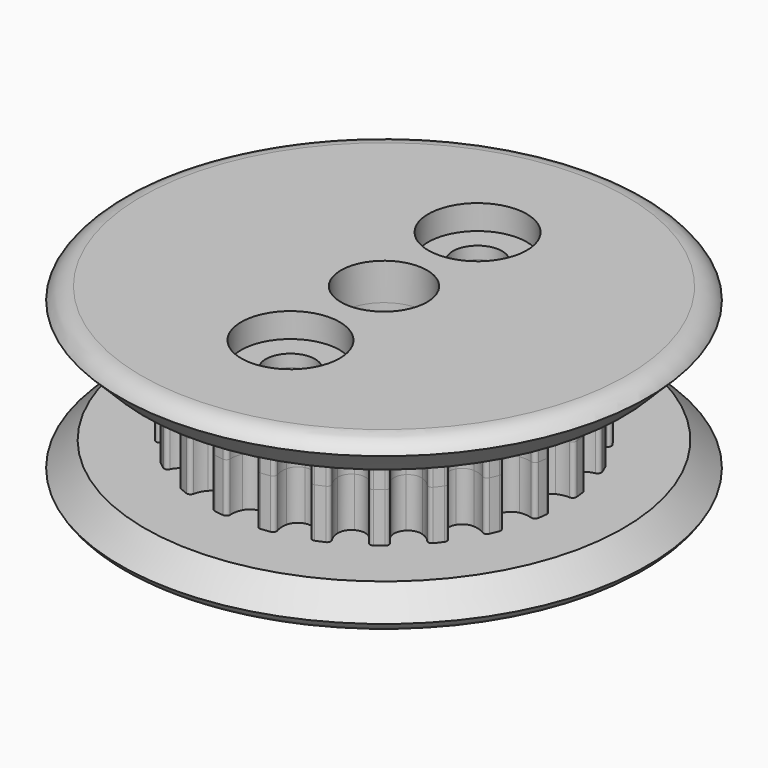
from build123d import *

# Parameters (mm, degrees)
F1_DEPTH      = 2
F1_DEPTH_BACK = 2
F4_SIZE       = 1
F4_2_SIZE     = 1
F6_R          = 1.75
F6_R_2        = 1
F7_DEPTH      = 7.001
F8_R          = 2
F9_DEPTH      = 1


# Not quite as in the source:
# - a fillet or chamfer that OpenCascade refuses, or shapes differently, is made with other operations: its cross-section is extruded or revolved along the edge and cut away or added


with BuildPart() as f1:
    # F0 (on Top) → F1 (new body, two sides)
    with BuildSketch(Plane.XY) as f1_sk:
        with BuildLine():
            ThreePointArc((-0.5986152965, 7.0620442035), (-0.6451801887, 7.1787658618), (-0.7641980304, 7.2191018018))
            ThreePointArc((-0.7641980304, 7.2191018018), (-0.9475467043, 7.1973317762), (-1.1302824209, 7.1709058774))
            ThreePointArc((-1.1302824209, 7.1709058774), (-1.2348051185, 7.1011402672), (-1.2495735623, 6.976343922))
            ThreePointArc((-1.2495735623, 6.976343922), (-1.2024254376, 6.7283466079), (-1.2188831701, 6.4764443322))
            ThreePointArc((-1.2188831701, 6.4764443322), (-1.3577692814, 6.2037699974), (-1.6200615767, 6.0461521156))
            ThreePointArc((-1.6200615767, 6.0461521156), (-1.9260223085, 6.0515070577), (-2.1826383766, 6.218206903))
            ThreePointArc((-2.1826383766, 6.218206903), (-2.3228423289, 6.4281318067), (-2.4060095121, 6.6664778432))
            ThreePointArc((-2.4060095121, 6.6664778432), (-2.4811975322, 6.7671704264), (-2.6065996488, 6.7753278684))
            ThreePointArc((-2.6065996488, 6.7753278684), (-2.7780663709, 6.7068455098), (-2.947735993, 6.634024568))
            ThreePointArc((-2.947735993, 6.634024568), (-3.0306404975, 6.5395836985), (-3.0126060479, 6.4152173311))
            ThreePointArc((-3.0126060479, 6.4152173311), (-2.9028780285, 6.1878731533), (-2.853577871, 5.9402946649))
            ThreePointArc((-2.853577871, 5.9402946649), (-2.9171582418, 5.6409651119), (-3.1297186342, 5.4208316878))
            ThreePointArc((-3.1297186342, 5.4208316878), (-3.4266399679, 5.3468157002), (-3.7176571503, 5.4414182604))
            ThreePointArc((-3.7176571503, 5.4414182604), (-3.9074163319, 5.6079026934), (-4.0494381556, 5.8166020346))
            ThreePointArc((-4.0494381556, 5.8166020346), (-4.1481253643, 5.8944035098), (-4.2713658087, 5.8698265376))
            ThreePointArc((-4.2713658087, 5.8698265376), (-4.4192654053, 5.7592988055), (-4.5643062286, 5.6450454476))
            ThreePointArc((-4.5643062286, 5.6450454476), (-4.6199427349, 5.5323653079), (-4.5703344099, 5.4169042808))
            ThreePointArc((-4.5703344099, 5.4169042808), (-4.4055042791, 5.2257063691), (-4.2938059557, 4.9993237329))
            ThreePointArc((-4.2938059557, 4.9993237329), (-4.2777476889, 4.6937377762), (-4.4260905389, 4.4260905389))
            ThreePointArc((-4.4260905389, 4.4260905389), (-4.6937377762, 4.2777476889), (-4.9993237329, 4.2938059557))
            ThreePointArc((-4.9993237329, 4.2938059557), (-5.2257063691, 4.4055042791), (-5.4169042808, 4.5703344099))
            ThreePointArc((-5.4169042808, 4.5703344099), (-5.5323653079, 4.6199427349), (-5.6450454476, 4.5643062286))
            ThreePointArc((-5.6450454476, 4.5643062286), (-5.7592988055, 4.4192654053), (-5.8698265376, 4.2713658087))
            ThreePointArc((-5.8698265376, 4.2713658087), (-5.8944035098, 4.1481253643), (-5.8166020346, 4.0494381556))
            ThreePointArc((-5.8166020346, 4.0494381556), (-5.6079026934, 3.9074163319), (-5.4414182604, 3.7176571503))
            ThreePointArc((-5.4414182604, 3.7176571503), (-5.3468157002, 3.4266399679), (-5.4208316878, 3.1297186342))
            ThreePointArc((-5.4208316878, 3.1297186342), (-5.6409651119, 2.9171582418), (-5.9402946649, 2.853577871))
            ThreePointArc((-5.9402946649, 2.853577871), (-6.1878731533, 2.9028780285), (-6.4152173311, 3.0126060479))
            ThreePointArc((-6.4152173311, 3.0126060479), (-6.5395836985, 3.0306404975), (-6.634024568, 2.947735993))
            ThreePointArc((-6.634024568, 2.947735993), (-6.7068455098, 2.7780663709), (-6.7753278684, 2.6065996488))
            ThreePointArc((-6.7753278684, 2.6065996488), (-6.7671704264, 2.4811975322), (-6.6664778432, 2.4060095121))
            ThreePointArc((-6.6664778432, 2.4060095121), (-6.4281318067, 2.3228423289), (-6.218206903, 2.1826383766))
            ThreePointArc((-6.218206903, 2.1826383766), (-6.0515070577, 1.9260223085), (-6.0461521156, 1.6200615767))
            ThreePointArc((-6.0461521156, 1.6200615767), (-6.2037699974, 1.3577692814), (-6.4764443322, 1.2188831701))
            ThreePointArc((-6.4764443322, 1.2188831701), (-6.7283466079, 1.2024254376), (-6.976343922, 1.2495735623))
            ThreePointArc((-6.976343922, 1.2495735623), (-7.1011402672, 1.2348051185), (-7.1709058774, 1.1302824209))
            ThreePointArc((-7.1709058774, 1.1302824209), (-7.1973317762, 0.9475467043), (-7.2191018018, 0.7641980304))
            ThreePointArc((-7.2191018018, 0.7641980304), (-7.1787658618, 0.6451801887), (-7.0620442035, 0.5986152965))
            ThreePointArc((-7.0620442035, 0.5986152965), (-6.8102943604, 0.5799704599), (-6.5712350212, 0.4988764045))
            ThreePointArc((-6.5712350212, 0.4988764045), (-6.3437982097, 0.2941494117), (-6.2594372684, 0))
            ThreePointArc((-6.2594372684, 0), (-6.3437982097, -0.2941494117), (-6.5712350212, -0.4988764045))
            ThreePointArc((-6.5712350212, -0.4988764045), (-6.8102943604, -0.5799704599), (-7.0620442035, -0.5986152965))
            ThreePointArc((-7.0620442035, -0.5986152965), (-7.1787658618, -0.6451801887), (-7.2191018018, -0.7641980304))
            ThreePointArc((-7.2191018018, -0.7641980304), (-7.1973317762, -0.9475467043), (-7.1709058774, -1.1302824209))
            ThreePointArc((-7.1709058774, -1.1302824209), (-7.1011402672, -1.2348051185), (-6.976343922, -1.2495735623))
            ThreePointArc((-6.976343922, -1.2495735623), (-6.7283466079, -1.2024254376), (-6.4764443322, -1.2188831701))
            ThreePointArc((-6.4764443322, -1.2188831701), (-6.2037699974, -1.3577692814), (-6.0461521156, -1.6200615767))
            ThreePointArc((-6.0461521156, -1.6200615767), (-6.0515070577, -1.9260223085), (-6.218206903, -2.1826383766))
            ThreePointArc((-6.218206903, -2.1826383766), (-6.4281318067, -2.3228423289), (-6.6664778432, -2.4060095121))
            ThreePointArc((-6.6664778432, -2.4060095121), (-6.7671704264, -2.4811975322), (-6.7753278684, -2.6065996488))
            ThreePointArc((-6.7753278684, -2.6065996488), (-6.7068455098, -2.7780663709), (-6.634024568, -2.947735993))
            ThreePointArc((-6.634024568, -2.947735993), (-6.5395836985, -3.0306404975), (-6.4152173311, -3.0126060479))
            ThreePointArc((-6.4152173311, -3.0126060479), (-6.1878731533, -2.9028780285), (-5.9402946649, -2.853577871))
            ThreePointArc((-5.9402946649, -2.853577871), (-5.6409651119, -2.9171582418), (-5.4208316878, -3.1297186342))
            ThreePointArc((-5.4208316878, -3.1297186342), (-5.3468157002, -3.4266399679), (-5.4414182604, -3.7176571503))
            ThreePointArc((-5.4414182604, -3.7176571503), (-5.6079026934, -3.9074163319), (-5.8166020346, -4.0494381556))
            ThreePointArc((-5.8166020346, -4.0494381556), (-5.8944035098, -4.1481253643), (-5.8698265376, -4.2713658087))
            ThreePointArc((-5.8698265376, -4.2713658087), (-5.7592988055, -4.4192654053), (-5.6450454476, -4.5643062286))
            ThreePointArc((-5.6450454476, -4.5643062286), (-5.5323653079, -4.6199427349), (-5.4169042808, -4.5703344099))
            ThreePointArc((-5.4169042808, -4.5703344099), (-5.2257063691, -4.4055042791), (-4.9993237329, -4.2938059557))
            ThreePointArc((-4.9993237329, -4.2938059557), (-4.6937377762, -4.2777476889), (-4.4260905389, -4.4260905389))
            ThreePointArc((-4.4260905389, -4.4260905389), (-4.2777476889, -4.6937377762), (-4.2938059557, -4.9993237329))
            ThreePointArc((-4.2938059557, -4.9993237329), (-4.4055042791, -5.2257063691), (-4.5703344099, -5.4169042808))
            ThreePointArc((-4.5703344099, -5.4169042808), (-4.6199427349, -5.5323653079), (-4.5643062286, -5.6450454476))
            ThreePointArc((-4.5643062286, -5.6450454476), (-4.4192654053, -5.7592988055), (-4.2713658087, -5.8698265376))
            ThreePointArc((-4.2713658087, -5.8698265376), (-4.1481253643, -5.8944035098), (-4.0494381556, -5.8166020346))
            ThreePointArc((-4.0494381556, -5.8166020346), (-3.9074163319, -5.6079026934), (-3.7176571503, -5.4414182604))
            ThreePointArc((-3.7176571503, -5.4414182604), (-3.4266399679, -5.3468157002), (-3.1297186342, -5.4208316878))
            ThreePointArc((-3.1297186342, -5.4208316878), (-2.9171582418, -5.6409651119), (-2.853577871, -5.9402946649))
            ThreePointArc((-2.853577871, -5.9402946649), (-2.9028780285, -6.1878731533), (-3.0126060479, -6.4152173311))
            ThreePointArc((-3.0126060479, -6.4152173311), (-3.0306404975, -6.5395836985), (-2.947735993, -6.634024568))
            ThreePointArc((-2.947735993, -6.634024568), (-2.7780663709, -6.7068455098), (-2.6065996488, -6.7753278684))
            ThreePointArc((-2.6065996488, -6.7753278684), (-2.4811975322, -6.7671704264), (-2.4060095121, -6.6664778432))
            ThreePointArc((-2.4060095121, -6.6664778432), (-2.3228423289, -6.4281318067), (-2.1826383766, -6.218206903))
            ThreePointArc((-2.1826383766, -6.218206903), (-1.9260223085, -6.0515070577), (-1.6200615767, -6.0461521156))
            ThreePointArc((-1.6200615767, -6.0461521156), (-1.3577692814, -6.2037699974), (-1.2188831701, -6.4764443322))
            ThreePointArc((-1.2188831701, -6.4764443322), (-1.2024254376, -6.7283466079), (-1.2495735623, -6.976343922))
            ThreePointArc((-1.2495735623, -6.976343922), (-1.2348051185, -7.1011402672), (-1.1302824209, -7.1709058774))
            ThreePointArc((-1.1302824209, -7.1709058774), (-0.9475467043, -7.1973317762), (-0.7641980304, -7.2191018018))
            ThreePointArc((-0.7641980304, -7.2191018018), (-0.6451801887, -7.1787658618), (-0.5986152965, -7.0620442035))
            ThreePointArc((-0.5986152965, -7.0620442035), (-0.5799704599, -6.8102943604), (-0.4988764045, -6.5712350212))
            ThreePointArc((-0.4988764045, -6.5712350212), (-0.2941494117, -6.3437982097), (0, -6.2594372684))
            ThreePointArc((0, -6.2594372684), (0.2941494117, -6.3437982097), (0.4988764045, -6.5712350212))
            ThreePointArc((0.4988764045, -6.5712350212), (0.5799704599, -6.8102943604), (0.5986152965, -7.0620442035))
            ThreePointArc((0.5986152965, -7.0620442035), (0.6451801887, -7.1787658618), (0.7641980304, -7.2191018018))
            ThreePointArc((0.7641980304, -7.2191018018), (0.9475467043, -7.1973317762), (1.1302824209, -7.1709058774))
            ThreePointArc((1.1302824209, -7.1709058774), (1.2348051185, -7.1011402672), (1.2495735623, -6.976343922))
            ThreePointArc((1.2495735623, -6.976343922), (1.2024254376, -6.7283466079), (1.2188831701, -6.4764443322))
            ThreePointArc((1.2188831701, -6.4764443322), (1.3577692814, -6.2037699974), (1.6200615767, -6.0461521156))
            ThreePointArc((1.6200615767, -6.0461521156), (1.9260223085, -6.0515070577), (2.1826383766, -6.218206903))
            ThreePointArc((2.1826383766, -6.218206903), (2.3228423289, -6.4281318067), (2.4060095121, -6.6664778432))
            ThreePointArc((2.4060095121, -6.6664778432), (2.4811975322, -6.7671704264), (2.6065996488, -6.7753278684))
            ThreePointArc((2.6065996488, -6.7753278684), (2.7780663709, -6.7068455098), (2.947735993, -6.634024568))
            ThreePointArc((2.947735993, -6.634024568), (3.0306404975, -6.5395836985), (3.0126060479, -6.4152173311))
            ThreePointArc((3.0126060479, -6.4152173311), (2.9028780285, -6.1878731533), (2.853577871, -5.9402946649))
            ThreePointArc((2.853577871, -5.9402946649), (2.9171582418, -5.6409651119), (3.1297186342, -5.4208316878))
            ThreePointArc((3.1297186342, -5.4208316878), (3.4266399679, -5.3468157002), (3.7176571503, -5.4414182604))
            ThreePointArc((3.7176571503, -5.4414182604), (3.9074163319, -5.6079026934), (4.0494381556, -5.8166020346))
            ThreePointArc((4.0494381556, -5.8166020346), (4.1481253643, -5.8944035098), (4.2713658087, -5.8698265376))
            ThreePointArc((4.2713658087, -5.8698265376), (4.4192654053, -5.7592988055), (4.5643062286, -5.6450454476))
            ThreePointArc((4.5643062286, -5.6450454476), (4.6199427349, -5.5323653079), (4.5703344099, -5.4169042808))
            ThreePointArc((4.5703344099, -5.4169042808), (4.4055042791, -5.2257063691), (4.2938059557, -4.9993237329))
            ThreePointArc((4.2938059557, -4.9993237329), (4.2777476889, -4.6937377762), (4.4260905389, -4.4260905389))
            ThreePointArc((4.4260905389, -4.4260905389), (4.6937377762, -4.2777476889), (4.9993237329, -4.2938059557))
            ThreePointArc((4.9993237329, -4.2938059557), (5.2257063691, -4.4055042791), (5.4169042808, -4.5703344099))
            ThreePointArc((5.4169042808, -4.5703344099), (5.5323653079, -4.6199427349), (5.6450454476, -4.5643062286))
            ThreePointArc((5.6450454476, -4.5643062286), (5.7592988055, -4.4192654053), (5.8698265376, -4.2713658087))
            ThreePointArc((5.8698265376, -4.2713658087), (5.8944035098, -4.1481253643), (5.8166020346, -4.0494381556))
            ThreePointArc((5.8166020346, -4.0494381556), (5.6079026934, -3.9074163319), (5.4414182604, -3.7176571503))
            ThreePointArc((5.4414182604, -3.7176571503), (5.3468157002, -3.4266399679), (5.4208316878, -3.1297186342))
            ThreePointArc((5.4208316878, -3.1297186342), (5.6409651119, -2.9171582418), (5.9402946649, -2.853577871))
            ThreePointArc((5.9402946649, -2.853577871), (6.1878731533, -2.9028780285), (6.4152173311, -3.0126060479))
            ThreePointArc((6.4152173311, -3.0126060479), (6.5395836985, -3.0306404975), (6.634024568, -2.947735993))
            ThreePointArc((6.634024568, -2.947735993), (6.7068455098, -2.7780663709), (6.7753278684, -2.6065996488))
            ThreePointArc((6.7753278684, -2.6065996488), (6.7671704264, -2.4811975322), (6.6664778432, -2.4060095121))
            ThreePointArc((6.6664778432, -2.4060095121), (6.4281318067, -2.3228423289), (6.218206903, -2.1826383766))
            ThreePointArc((6.218206903, -2.1826383766), (6.0515070577, -1.9260223085), (6.0461521156, -1.6200615767))
            ThreePointArc((6.0461521156, -1.6200615767), (6.2037699974, -1.3577692814), (6.4764443322, -1.2188831701))
            ThreePointArc((6.4764443322, -1.2188831701), (6.7283466079, -1.2024254376), (6.976343922, -1.2495735623))
            ThreePointArc((6.976343922, -1.2495735623), (7.1011402672, -1.2348051185), (7.1709058774, -1.1302824209))
            ThreePointArc((7.1709058774, -1.1302824209), (7.1973317762, -0.9475467043), (7.2191018018, -0.7641980304))
            ThreePointArc((7.2191018018, -0.7641980304), (7.1787658618, -0.6451801887), (7.0620442035, -0.5986152965))
            ThreePointArc((7.0620442035, -0.5986152965), (6.8102943604, -0.5799704599), (6.5712350212, -0.4988764045))
            ThreePointArc((6.5712350212, -0.4988764045), (6.3437982097, -0.2941494117), (6.2594372684, 0))
            ThreePointArc((6.2594372684, 0), (6.3437982097, 0.2941494117), (6.5712350212, 0.4988764045))
            ThreePointArc((6.5712350212, 0.4988764045), (6.8102943604, 0.5799704599), (7.0620442035, 0.5986152965))
            ThreePointArc((7.0620442035, 0.5986152965), (7.1787658618, 0.6451801887), (7.2191018018, 0.7641980304))
            ThreePointArc((7.2191018018, 0.7641980304), (7.1973317762, 0.9475467043), (7.1709058774, 1.1302824209))
            ThreePointArc((7.1709058774, 1.1302824209), (7.1011402672, 1.2348051185), (6.976343922, 1.2495735623))
            ThreePointArc((6.976343922, 1.2495735623), (6.7283466079, 1.2024254376), (6.4764443322, 1.2188831701))
            ThreePointArc((6.4764443322, 1.2188831701), (6.2037699974, 1.3577692814), (6.0461521156, 1.6200615767))
            ThreePointArc((6.0461521156, 1.6200615767), (6.0515070577, 1.9260223085), (6.218206903, 2.1826383766))
            ThreePointArc((6.218206903, 2.1826383766), (6.4281318067, 2.3228423289), (6.6664778432, 2.4060095121))
            ThreePointArc((6.6664778432, 2.4060095121), (6.7671704264, 2.4811975322), (6.7753278684, 2.6065996488))
            ThreePointArc((6.7753278684, 2.6065996488), (6.7068455098, 2.7780663709), (6.634024568, 2.947735993))
            ThreePointArc((6.634024568, 2.947735993), (6.5395836985, 3.0306404975), (6.4152173311, 3.0126060479))
            ThreePointArc((6.4152173311, 3.0126060479), (6.1878731533, 2.9028780285), (5.9402946649, 2.853577871))
            ThreePointArc((5.9402946649, 2.853577871), (5.6409651119, 2.9171582418), (5.4208316878, 3.1297186342))
            ThreePointArc((5.4208316878, 3.1297186342), (5.3468157002, 3.4266399679), (5.4414182604, 3.7176571503))
            ThreePointArc((5.4414182604, 3.7176571503), (5.6079026934, 3.9074163319), (5.8166020346, 4.0494381556))
            ThreePointArc((5.8166020346, 4.0494381556), (5.8944035098, 4.1481253643), (5.8698265376, 4.2713658087))
            ThreePointArc((5.8698265376, 4.2713658087), (5.7592988055, 4.4192654053), (5.6450454476, 4.5643062286))
            ThreePointArc((5.6450454476, 4.5643062286), (5.5323653079, 4.6199427349), (5.4169042808, 4.5703344099))
            ThreePointArc((5.4169042808, 4.5703344099), (5.2257063691, 4.4055042791), (4.9993237329, 4.2938059557))
            ThreePointArc((4.9993237329, 4.2938059557), (4.6937377762, 4.2777476889), (4.4260905389, 4.4260905389))
            ThreePointArc((4.4260905389, 4.4260905389), (4.2777476889, 4.6937377762), (4.2938059557, 4.9993237329))
            ThreePointArc((4.2938059557, 4.9993237329), (4.4055042791, 5.2257063691), (4.5703344099, 5.4169042808))
            ThreePointArc((4.5703344099, 5.4169042808), (4.6199427349, 5.5323653079), (4.5643062286, 5.6450454476))
            ThreePointArc((4.5643062286, 5.6450454476), (4.4192654053, 5.7592988055), (4.2713658087, 5.8698265376))
            ThreePointArc((4.2713658087, 5.8698265376), (4.1481253643, 5.8944035098), (4.0494381556, 5.8166020346))
            ThreePointArc((4.0494381556, 5.8166020346), (3.9074163319, 5.6079026934), (3.7176571503, 5.4414182604))
            ThreePointArc((3.7176571503, 5.4414182604), (3.4266399679, 5.3468157002), (3.1297186342, 5.4208316878))
            ThreePointArc((3.1297186342, 5.4208316878), (2.9171582418, 5.6409651119), (2.853577871, 5.9402946649))
            ThreePointArc((2.853577871, 5.9402946649), (2.9028780285, 6.1878731533), (3.0126060479, 6.4152173311))
            ThreePointArc((3.0126060479, 6.4152173311), (3.0306404975, 6.5395836985), (2.947735993, 6.634024568))
            ThreePointArc((2.947735993, 6.634024568), (2.7780663709, 6.7068455098), (2.6065996488, 6.7753278684))
            ThreePointArc((2.6065996488, 6.7753278684), (2.4811975322, 6.7671704264), (2.4060095121, 6.6664778432))
            ThreePointArc((2.4060095121, 6.6664778432), (2.3228423289, 6.4281318067), (2.1826383766, 6.218206903))
            ThreePointArc((2.1826383766, 6.218206903), (1.9260223085, 6.0515070577), (1.6200615767, 6.0461521156))
            ThreePointArc((1.6200615767, 6.0461521156), (1.3577692814, 6.2037699974), (1.2188831701, 6.4764443322))
            ThreePointArc((1.2188831701, 6.4764443322), (1.2024254376, 6.7283466079), (1.2495735623, 6.976343922))
            ThreePointArc((1.2495735623, 6.976343922), (1.2348051185, 7.1011402672), (1.1302824209, 7.1709058774))
            ThreePointArc((1.1302824209, 7.1709058774), (0.9475467043, 7.1973317762), (0.7641980304, 7.2191018018))
            ThreePointArc((0.7641980304, 7.2191018018), (0.6451801887, 7.1787658618), (0.5986152965, 7.0620442035))
            ThreePointArc((0.5986152965, 7.0620442035), (0.5799704599, 6.8102943604), (0.4988764045, 6.5712350212))
            ThreePointArc((0.4988764045, 6.5712350212), (0.2941494117, 6.3437982097), (0, 6.2594372684))
            ThreePointArc((0, 6.2594372684), (-0.2941494117, 6.3437982097), (-0.4988764045, 6.5712350212))
            ThreePointArc((-0.4988764045, 6.5712350212), (-0.5799704599, 6.8102943604), (-0.5986152965, 7.0620442035))
        make_face()
    extrude(amount=F1_DEPTH)
    extrude(f1_sk.sketch, amount=-F1_DEPTH_BACK)


with BuildPart() as f3:
    # F2 (on Right) → F3 (revolve)
    with BuildSketch(Plane.YZ):
        Polygon((0, 3.5), (0, 2), (7.2191018018, 2), (10.7191018018, 2), (10.7191018018, 3.5), align=None)
    revolve(axis=Axis((0, 0, 2.75), (0, 0, -1)))

    # F4
    f4_edges = [f3.edges().sort_by_distance(p)[0] for p in [
        (0, -10.719102, 2),
    ]]
    chamfer(f4_edges, length=F4_SIZE)

    # F5: fillet of radius 1 on 1 edges, made by hand

    # F5_s1 → F5_t2 (revolve, cut)
    with BuildSketch(Plane.YZ):
        with BuildLine():
            ThreePointArc((10.7191018018, 3), (10.353076398, 3.3660254038), (9.853076398, 3.5))
            Line((9.853076398, 3.5), (10.7191018018, 3.5))
            Line((10.7191018018, 3.5), (10.7191018018, 3))
        make_face()
    revolve(axis=Axis((0, 0, 3.5), (0, 0, -1)), mode=Mode.SUBTRACT)


with BuildPart() as f3b:
    # F2 (on Right) → F3, piece 2 (revolve)
    with BuildSketch(Plane.YZ):
        Polygon((0, -2), (0, -3.5), (10.7191018018, -3.5), (10.7191018018, -2), (7.2191018018, -2), align=None)
    revolve(axis=Axis((0, 0, 2.75), (0, 0, -1)))

    # F4#2
    f4_2_edges = [f3b.edges().sort_by_distance(p)[0] for p in [
        (0, -10.719102, -2),
    ]]
    chamfer(f4_2_edges, length=F4_2_SIZE)

    # F5#2: fillet of radius 1 on 1 edges, made by hand

    # F5_2_s1 → F5_2_t2 (revolve, cut)
    with BuildSketch(Plane.YZ):
        with BuildLine():
            ThreePointArc((10.7191018018, -3), (10.353076398, -3.3660254038), (9.853076398, -3.5))
            Line((9.853076398, -3.5), (10.7191018018, -3.5))
            Line((10.7191018018, -3.5), (10.7191018018, -3))
        make_face()
    revolve(axis=Axis((0, 0, -3.5), (0, 0, -1)), mode=Mode.SUBTRACT)


with BuildPart() as f7_tool:
    # F6 (on face) → F7 (new body, through all)
    with BuildSketch(Plane.XY.offset(3.5)):
        Circle(F6_R)
        with Locations((0, -4.75)):
            Circle(F6_R_2)
        with Locations((0, 4.75)):
            Circle(F6_R_2)
    extrude(amount=-F7_DEPTH)


with BuildPart() as f1_1:
    add(f1.part)

    # F7: cut by f7_tool
    add(f7_tool.part, mode=Mode.SUBTRACT)


with BuildPart() as f3_1:
    add(f3.part)

    # F7: cut by f7_tool
    add(f7_tool.part, mode=Mode.SUBTRACT)

    # F8 (on face) → F9 (cut)
    with BuildSketch(Plane.XY.offset(3.5)):
        with Locations((0, 4.75)):
            Circle(F8_R)
        with Locations((0, -4.75)):
            Circle(F8_R)
    extrude(amount=-F9_DEPTH, mode=Mode.SUBTRACT)


with BuildPart() as f3b_1:
    add(f3b.part)

    # F7: cut by f7_tool
    add(f7_tool.part, mode=Mode.SUBTRACT)


solid = Compound([f1_1.part, f3_1.part, f3b_1.part])
